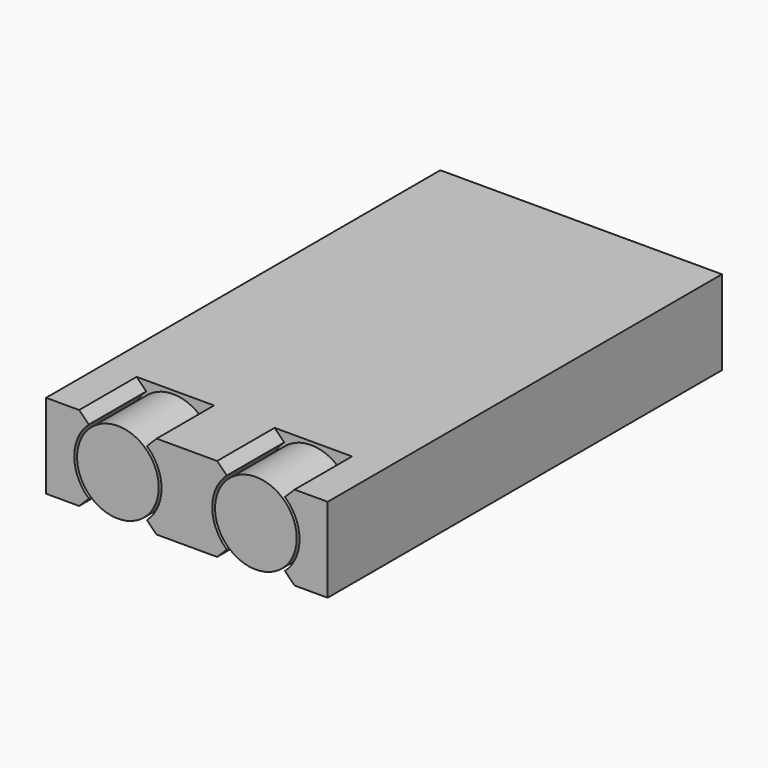
from build123d import *

# Parameters (mm, degrees)
F0_W        = 20
F0_H        = 6
F1_DEPTH    = 35
F3_DEPTH    = 5.1
F4_T1_DEPTH = 7.671682988
F7_R        = 2.9
F8_DEPTH    = 4.9
F5_R        = 1.5
F9_DEPTH    = 10


# Not quite as in the source:
# - a fillet or chamfer that OpenCascade refuses, or shapes differently, is made with other operations: its cross-section is extruded or revolved along the edge and cut away or added


with BuildPart() as f1:
    # F0 (on Front) → F1 (new body)
    with BuildSketch(Plane.XZ):
        Rectangle(F0_W, F0_H)
    extrude(amount=F1_DEPTH)

    # F2 (on face) → F3 (cut)
    with BuildSketch(Plane.XZ.offset(35)):
        with BuildLine():
            Line((-6.65, 3.1), (-6.65, 2.5588083164))
            ThreePointArc((-6.65, 2.5588083164), (-8, 0), (-6.65, -2.5588083164))
            Line((-6.65, -2.5588083164), (-6.65, -3.1))
            Line((-6.65, -3.1), (-3.15, -3.1))
            Line((-3.15, -3.1), (-3.15, -2.5588083164))
            ThreePointArc((-3.15, -2.5588083164), (-1.8, 0), (-3.15, 2.5588083164))
            Line((-3.15, 2.5588083164), (-3.15, 3.1))
            Line((-3.15, 3.1), (-6.65, 3.1))
        make_face()
        with BuildLine():
            Line((6.65, -3.1), (6.65, -2.5588083164))
            ThreePointArc((6.65, -2.5588083164), (8, 0), (6.65, 2.5588083164))
            Line((6.65, 2.5588083164), (6.65, 3.1))
            Line((6.65, 3.1), (3.15, 3.1))
            Line((3.15, 3.1), (3.15, 2.5588083164))
            ThreePointArc((3.15, 2.5588083164), (1.8, 0), (3.15, -2.5588083164))
            Line((3.15, -2.5588083164), (3.15, -3.1))
            Line((3.15, -3.1), (6.65, -3.1))
        make_face()
    extrude(amount=-F3_DEPTH, mode=Mode.SUBTRACT)

    # F4: chamfer of 1 on 8 edges, made by hand

    # F4_s2 → F4_t1 (cut)
    with BuildSketch(Plane.XZ.offset(29.9)):
        Polygon((-7.65, 3), (-6.65, 2), (-6.65, 3), align=None)
        Polygon((-2.15, 3), (-3.15, 2), (-3.15, 3), align=None)
        Polygon((2.15, 3), (3.15, 2), (3.15, 3), align=None)
        Polygon((7.65, 3), (6.65, 2), (6.65, 3), align=None)
        Polygon((-7.65, -3), (-6.65, -2), (-6.65, -3), align=None)
        Polygon((-2.15, -3), (-3.15, -2), (-3.15, -3), align=None)
        Polygon((2.15, -3), (3.15, -2), (3.15, -3), align=None)
        Polygon((7.65, -3), (6.65, -2), (6.65, -3), align=None)
    extrude(amount=F4_T1_DEPTH, mode=Mode.SUBTRACT)

    # F5 (on face) → F9 (cut)
    with BuildSketch(Plane(origin=(0, 0, 0), x_dir=(-1, 0, 0), z_dir=(0, 1, 0))):
        with Locations((-6.5, 0)):
            Circle(F5_R)
        with Locations((6.5, 0)):
            Circle(F5_R)
    extrude(amount=-F9_DEPTH, mode=Mode.SUBTRACT)


with BuildPart() as f8:
    # F7 (on offset) → F8 (new body)
    with BuildSketch(Plane.XZ.offset(30.1)):
        with Locations((-4.9, 0)):
            Circle(F7_R)
    extrude(amount=F8_DEPTH)


with BuildPart() as f8b:
    # F7 (on offset) → F8, piece 2 (new body)
    with BuildSketch(Plane.XZ.offset(30.1)):
        with Locations((4.9, 0)):
            Circle(F7_R)
    extrude(amount=F8_DEPTH)


solid = Compound([f1.part, f8.part, f8b.part])
